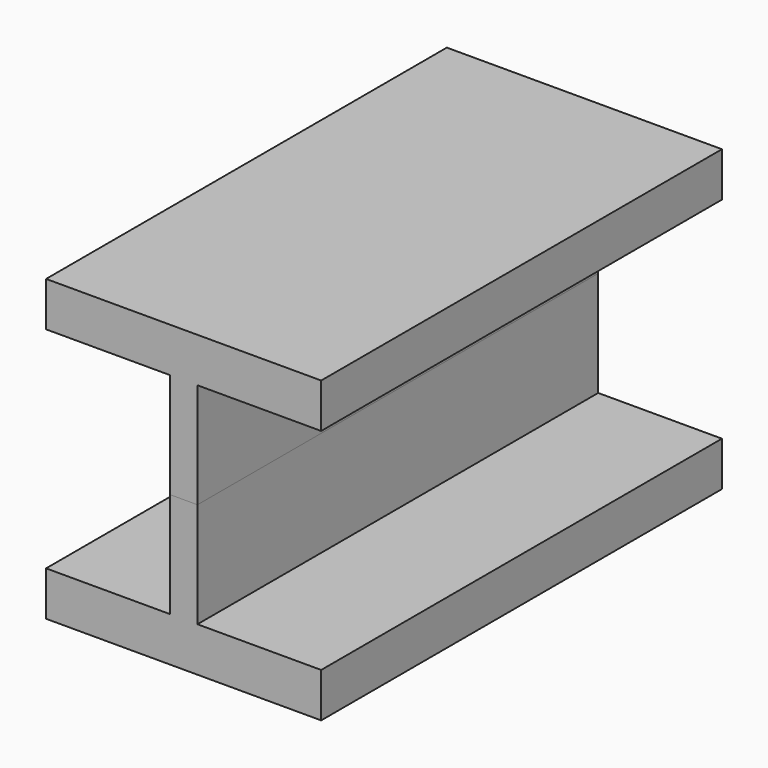
from build123d import *

# Parameters (mm, degrees)
F0_W     = 188.214
F0_H     = 67.564
F0_W_2   = 21.0185
F0_H_2   = 160.02
F1_DEPTH = 762


# Not quite as in the source:
# - a pattern or mirror of a feature is missing from the dataset's text; its kind, count and spacing are read off the source's solid


with BuildPart() as f1:
    # F0 (on Front) → F1 (new body)
    with BuildSketch(Plane.XZ):
        with Locations((115.1255, 0)):
            Rectangle(F0_W, F0_H)
        Polygon((21.0185, -33.782), (21.0185, 33.782), (0, 33.782), (0, 0), (0, -33.782), align=None)
        with Locations((10.50925, 113.792)):
            Rectangle(F0_W_2, F0_H_2)
        Polygon((0, 0), (0, 33.782), (-21.0185, 33.782), (-21.0185, -33.782), (0, -33.782), align=None)
        with Locations((-10.50925, 113.792)):
            Rectangle(F0_W_2, F0_H_2)
        with Locations((-115.1255, 0)):
            Rectangle(F0_W, F0_H)
    extrude(amount=F1_DEPTH)


with BuildPart() as f1_copies_1:
    # F1_copies: instance of F1
    add(f1.part.mirror(Plane.XY.offset(193.802)))


solid = Compound([f1.part, f1_copies_1.part])
